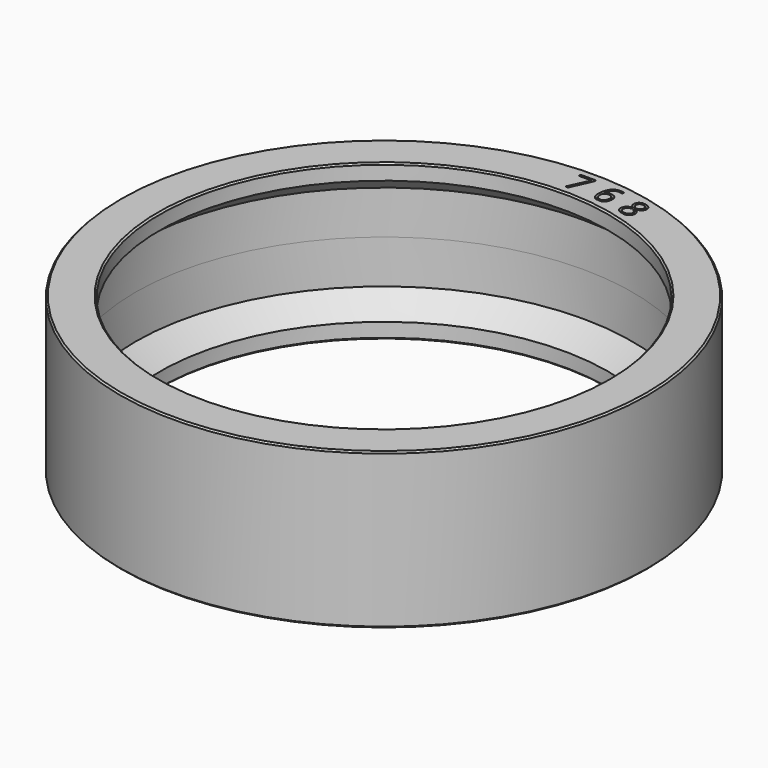
from build123d import *

# Parameters (mm, degrees)
F0_R          = 17
F0_R_2        = 16
F0_R_3        = 14.45
F1_DEPTH      = 5
F2_DEPTH      = 4
F2_DEPTH_BACK = 4
F3_SIZE2      = 1.19999
F3_SIZE       = 1.54999
F4_SIZE       = 0.1
F5_TEXT_SIZE  = 2.0833333333
F6_DEPTH      = 0.2
F7_SIZE       = 0.1


# Not quite as in the source:
# - a fillet or chamfer is up to 0.001 mm smaller than in the source, because OpenCascade refuses the exact size
# - Text() gives the source's letters only with a copy of the font that has no kerning and outlines rounded to 1/6400 em; it was checked with that copy


with BuildPart() as f1:
    # F0 (on Top) → F1 (new body, symmetric)
    with BuildSketch(Plane.XY):
        Circle(F0_R)
        Circle(F0_R_2, mode=Mode.SUBTRACT)
        Circle(F0_R_2)
        Circle(F0_R_3, mode=Mode.SUBTRACT)
    extrude(amount=F1_DEPTH, both=True)

    # F0 (on Top) → F2 (cut, two sides)
    with BuildSketch(Plane.XY) as f2_sk:
        Circle(F0_R_2)
        Circle(F0_R_3, mode=Mode.SUBTRACT)
    extrude(amount=F2_DEPTH, mode=Mode.SUBTRACT)
    extrude(f2_sk.sketch, amount=-F2_DEPTH_BACK, mode=Mode.SUBTRACT)

    # F3 (size 1.55 and 1.2 in the source; OpenCascade refuses exactly that, so slightly less here)
    f3_edges = [f1.edges().sort_by_distance(p)[0] for p in [
        (-16, 0, -4),
        (-16, 0, 4),
    ]]
    chamfer(f3_edges, length=F3_SIZE, length2=F3_SIZE2)

    # F4
    f4_edges = [f1.edges().sort_by_distance(p)[0] for p in [
        (-17, 0, 5),
        (-17, 0, -5),
    ]]
    chamfer(f4_edges, length=F4_SIZE)

    # F5 (on face) → F6 (cut)
    with BuildSketch(Plane.XY.offset(5)):
        with BuildLine():
            add(Edge.make_bspline(
                [(1.7640583925, 14.8640148532), (1.6221336106, 14.9170469744), (1.5409525768, 15.0535640714)],
                knots=[0.2780169607, 0.2780169607, 0.2780169607, 1, 1, 1], degree=2))
            Line((1.7640583925, 14.8640148532), (1.8768651726, 14.8569176522))
            Line((1.8768651726, 14.8569176522), (2.0058574013, 14.8323110686))
            add(Edge.make_bspline(
                [(2.2387621449, 14.9243967145), (2.1397181269, 14.8437172462), (2.0058574013, 14.8323110686)],
                knots=[0, 0, 0, 0.6961452699, 0.6961452699, 0.6961452699], degree=2))
            add(Edge.make_bspline(
                [(2.4101264593, 15.2705575063), (2.3810370727, 15.0402913012), (2.2387621449, 14.9243967145)],
                knots=[0, 0, 0, 1, 1, 1], degree=2))
            add(Edge.make_bspline(
                [(2.3368050306, 15.6108811928), (2.4361151538, 15.476279207), (2.4101264593, 15.2705575063)],
                knots=[0, 0, 0, 1, 1, 1], degree=2))
            add(Edge.make_bspline(
                [(2.0385552406, 15.7706151029), (2.2374949073, 15.7454831785), (2.3368050306, 15.6108811928)],
                knots=[0, 0, 0, 1, 1, 1], degree=2))
            add(Edge.make_bspline(
                [(1.6652316486, 15.6412547022), (1.7982774614, 15.8009692454), (2.0385552406, 15.7706151029)],
                knots=[0, 0, 0, 1, 1, 1], degree=2))
            Line((1.6652316486, 15.6412547022), (1.6532823504, 15.6427642496))
            add(Edge.make_bspline(
                [(1.8491058792, 16.0903375422), (1.7052958528, 15.9583955344), (1.6532823504, 15.6427642496)],
                knots=[0, 0, 0, 1, 1, 1], degree=2))
            add(Edge.make_bspline(
                [(2.2302870988, 16.1922925946), (1.9929159056, 16.2222795499), (1.8491058792, 16.0903375422)],
                knots=[0, 0, 0, 1, 1, 1], degree=2))
            add(Edge.make_bspline(
                [(2.4047295121, 16.1446629641), (2.3300798861, 16.1796858338), (2.2302870988, 16.1922925946)],
                knots=[0, 0, 0, 1, 1, 1], degree=2))
            Line((2.4047295121, 16.1446629641), (2.4229664767, 16.289023404))
            add(Edge.make_bspline(
                [(2.2458111664, 16.3307617), (2.35981393, 16.3163598017), (2.4229664767, 16.289023404)],
                knots=[0, 0, 0, 1, 1, 1], degree=2))
            add(Edge.make_bspline(
                [(1.7185042388, 16.1785279781), (1.914783312, 16.3725802431), (2.2458111664, 16.3307617)],
                knots=[0, 0, 0, 1, 1, 1], degree=2))
            add(Edge.make_bspline(
                [(1.4672694801, 15.5494566693), (1.5222251656, 15.9844757131), (1.7185042388, 16.1785279781)],
                knots=[0, 0, 0, 1, 1, 1], degree=2))
            add(Edge.make_bspline(
                [(1.5409525768, 15.0535640714), (1.4285108304, 15.2426503652), (1.4672694801, 15.5494566693)],
                knots=[0, 0, 0, 1, 1, 1], degree=2))
        make_face()
        with BuildLine():
            add(Edge.make_bspline(
                [(1.8984231614, 14.9782190928), (2.0418147394, 14.9601045239), (2.1323620724, 15.0405359934)],
                knots=[0, 0, 0, 1, 1, 1], degree=2))
            add(Edge.make_bspline(
                [(1.7359865092, 15.0520571744), (1.8034746842, 14.9902138749), (1.8984231614, 14.9782190928)],
                knots=[0, 0, 0, 1, 1, 1], degree=2))
            add(Edge.make_bspline(
                [(1.6394710885, 15.2087815095), (1.6684983342, 15.1139004739), (1.7359865092, 15.0520571744)],
                knots=[0, 0, 0, 1, 1, 1], degree=2))
            add(Edge.make_bspline(
                [(1.6235809852, 15.4076537344), (1.6104438429, 15.303662545), (1.6394710885, 15.2087815095)],
                knots=[0, 0, 0, 1, 1, 1], degree=2))
            add(Edge.make_bspline(
                [(1.685688592, 15.5382693218), (1.6325158739, 15.4783806614), (1.6235809852, 15.4076537344)],
                knots=[0, 0, 0, 1, 1, 1], degree=2))
            add(Edge.make_bspline(
                [(1.8193266592, 15.6260533801), (1.73886131, 15.5981579823), (1.685688592, 15.5382693218)],
                knots=[0, 0, 0, 1, 1, 1], degree=2))
            add(Edge.make_bspline(
                [(1.9905420835, 15.6424843773), (1.8997920083, 15.6539487779), (1.8193266592, 15.6260533801)],
                knots=[0, 0, 0, 1, 1, 1], degree=2))
            add(Edge.make_bspline(
                [(2.1998865293, 15.5308939811), (2.1368402475, 15.6240026212), (1.9905420835, 15.6424843773)],
                knots=[0, 0, 0, 1, 1, 1], degree=2))
            add(Edge.make_bspline(
                [(2.244451055, 15.2914871771), (2.2629328112, 15.4377853411), (2.1998865293, 15.5308939811)],
                knots=[0, 0, 0, 1, 1, 1], degree=2))
            add(Edge.make_bspline(
                [(2.1323620724, 15.0405359934), (2.2229094055, 15.1209674628), (2.244451055, 15.2914871771)],
                knots=[0, 0, 0, 1, 1, 1], degree=2))
        make_face(mode=Mode.SUBTRACT)
        with Locations((-0.6101888021, 14.975)):
            Text('7', F5_TEXT_SIZE, font='Open Sans', text_align=(TextAlign.LEFT, TextAlign.BOTTOM))
        with BuildLine():
            add(Edge.make_bspline(
                [(3.5748231145, 14.5330148518), (3.4480209197, 14.5891704234), (3.3816003157, 14.6790202269)],
                knots=[0.3241707912, 0.3241707912, 0.3241707912, 1, 1, 1], degree=2))
            Line((3.5748231145, 14.5330148518), (3.7241310603, 14.5045328379))
            Line((3.7241310603, 14.5045328379), (3.8483350435, 14.4641765174))
            add(Edge.make_bspline(
                [(4.0805687598, 14.5059411415), (3.9788569504, 14.4560340761), (3.8483350435, 14.4641765174)],
                knots=[0, 0, 0, 0.666283244, 0.666283244, 0.666283244], degree=2))
            add(Edge.make_bspline(
                [(4.2792059954, 14.7599318099), (4.2332242715, 14.5808448192), (4.0805687598, 14.5059411415)],
                knots=[0, 0, 0, 1, 1, 1], degree=2))
            add(Edge.make_bspline(
                [(4.2600752344, 14.9923694983), (4.310373185, 14.8813199991), (4.2792059954, 14.7599318099)],
                knots=[0, 0, 0, 1, 1, 1], degree=2))
            add(Edge.make_bspline(
                [(4.0560075157, 15.23229748), (4.2097772838, 15.1034189975), (4.2600752344, 14.9923694983)],
                knots=[0, 0, 0, 1, 1, 1], degree=2))
            add(Edge.make_bspline(
                [(4.3079017923, 15.3376781912), (4.2195002073, 15.2669457914), (4.0560075157, 15.23229748)],
                knots=[0, 0, 0, 1, 1, 1], degree=2))
            add(Edge.make_bspline(
                [(4.4236657413, 15.5149799624), (4.3963033774, 15.4084105911), (4.3079017923, 15.3376781912)],
                knots=[0, 0, 0, 1, 1, 1], degree=2))
            add(Edge.make_bspline(
                [(4.3733911609, 15.7975919873), (4.4651140558, 15.6764104892), (4.4236657413, 15.5149799624)],
                knots=[0, 0, 0, 1, 1, 1], degree=2))
            add(Edge.make_bspline(
                [(4.0846095174, 15.9693695724), (4.281668266, 15.9187734853), (4.3733911609, 15.7975919873)],
                knots=[0, 0, 0, 1, 1, 1], degree=2))
            add(Edge.make_bspline(
                [(3.7507941645, 15.9559353688), (3.8903884147, 16.0192370758), (4.0846095174, 15.9693695724)],
                knots=[0, 0, 0, 1, 1, 1], degree=2))
            add(Edge.make_bspline(
                [(3.5709659058, 15.7359325449), (3.6111999142, 15.8926336618), (3.7507941645, 15.9559353688)],
                knots=[0, 0, 0, 1, 1, 1], degree=2))
            add(Edge.make_bspline(
                [(3.5788398134, 15.5211726182), (3.542632097, 15.6255796457), (3.5709659058, 15.7359325449)],
                knots=[0, 0, 0, 1, 1, 1], degree=2))
            add(Edge.make_bspline(
                [(3.7312674841, 15.3052580876), (3.6150475297, 15.4167655907), (3.5788398134, 15.5211726182)],
                knots=[0, 0, 0, 1, 1, 1], degree=2))
            add(Edge.make_bspline(
                [(3.3309209528, 14.9973605971), (3.3943886844, 15.2445510914), (3.7312674841, 15.3052580876)],
                knots=[0, 0, 0, 1, 1, 1], degree=2))
            add(Edge.make_bspline(
                [(3.3816003157, 14.6790202269), (3.2833201541, 14.8119677265), (3.3309209528, 14.9973605971)],
                knots=[0, 0, 0, 1, 1, 1], degree=2))
        make_face()
        with BuildLine():
            add(Edge.make_bspline(
                [(3.491614375, 14.9517325069), (3.4612567228, 14.8334972577), (3.5264310008, 14.7463547161)],
                knots=[0, 0, 0, 1, 1, 1], degree=2))
            add(Edge.make_bspline(
                [(3.6044639894, 15.1176836941), (3.5189767389, 15.0583018781), (3.491614375, 14.9517325069)],
                knots=[0, 0, 0, 1, 1, 1], degree=2))
            add(Edge.make_bspline(
                [(3.8530689906, 15.2023998671), (3.6899512398, 15.17706551), (3.6044639894, 15.1176836941)],
                knots=[0, 0, 0, 1, 1, 1], degree=2))
            add(Edge.make_bspline(
                [(4.0839920761, 14.9891845377), (4.0261654231, 15.0833466335), (3.8530689906, 15.2023998671)],
                knots=[0, 0, 0, 1, 1, 1], degree=2))
            add(Edge.make_bspline(
                [(4.1172897461, 14.7994883605), (4.1418187291, 14.8950224418), (4.0839920761, 14.9891845377)],
                knots=[0, 0, 0, 1, 1, 1], degree=2))
            add(Edge.make_bspline(
                [(3.9868987101, 14.6313194572), (4.0864463714, 14.6793613473), (4.1172897461, 14.7994883605)],
                knots=[0, 0, 0, 1, 1, 1], degree=2))
            add(Edge.make_bspline(
                [(3.7404240458, 14.6210020095), (3.8873510488, 14.583277567), (3.9868987101, 14.6313194572)],
                knots=[0, 0, 0, 1, 1, 1], degree=2))
            add(Edge.make_bspline(
                [(3.5264310008, 14.7463547161), (3.5916052789, 14.6592121745), (3.7404240458, 14.6210020095)],
                knots=[0, 0, 0, 1, 1, 1], degree=2))
        make_face(mode=Mode.SUBTRACT)
        with BuildLine():
            add(Edge.make_bspline(
                [(4.0486362291, 15.8371165218), (3.925356276, 15.8687694339), (3.8401821824, 15.8276235394)],
                knots=[0, 0, 0, 1, 1, 1], degree=2))
            add(Edge.make_bspline(
                [(4.2301646412, 15.7279971817), (4.1738079462, 15.8049778873), (4.0486362291, 15.8371165218)],
                knots=[0, 0, 0, 1, 1, 1], degree=2))
            add(Edge.make_bspline(
                [(4.2609399546, 15.5513835729), (4.2865213362, 15.6510164762), (4.2301646412, 15.7279971817)],
                knots=[0, 0, 0, 1, 1, 1], degree=2))
            add(Edge.make_bspline(
                [(4.1615755401, 15.4078480876), (4.2377062314, 15.4608941956), (4.2609399546, 15.5513835729)],
                knots=[0, 0, 0, 1, 1, 1], degree=2))
            add(Edge.make_bspline(
                [(3.9293700826, 15.3320283234), (4.0854448488, 15.3548019795), (4.1615755401, 15.4078480876)],
                knots=[0, 0, 0, 1, 1, 1], degree=2))
            add(Edge.make_bspline(
                [(3.7478906406, 15.5172570709), (3.789345436, 15.4372128954), (3.9293700826, 15.3320283234)],
                knots=[0, 0, 0, 1, 1, 1], degree=2))
            add(Edge.make_bspline(
                [(3.7296695684, 15.6877906237), (3.7064358452, 15.5973012463), (3.7478906406, 15.5172570709)],
                knots=[0, 0, 0, 1, 1, 1], degree=2))
            add(Edge.make_bspline(
                [(3.8401821824, 15.8276235394), (3.7550080888, 15.786477645), (3.7296695684, 15.6877906237)],
                knots=[0, 0, 0, 1, 1, 1], degree=2))
        make_face(mode=Mode.SUBTRACT)
    extrude(amount=-F6_DEPTH, mode=Mode.SUBTRACT)

    # F7
    f7_edges = [f1.edges().sort_by_distance(p)[0] for p in [
        (-14.45, 0, 5),
        (-14.45, 0, -5),
    ]]
    chamfer(f7_edges, length=F7_SIZE)


solid = f1.part
